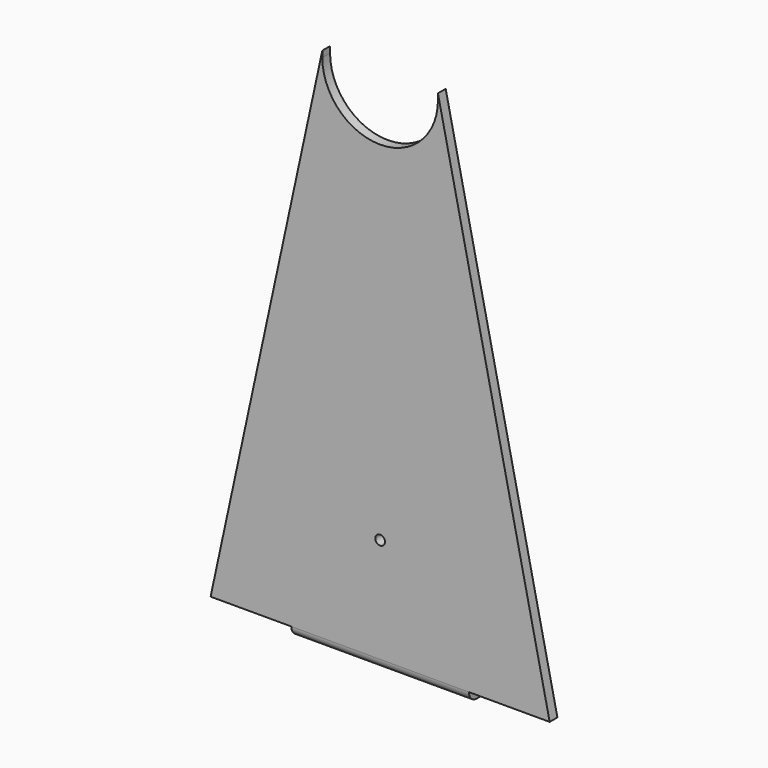
from build123d import *

# Parameters (mm, degrees)
F0_R     = 1.5
F1_DEPTH = 3
F2_W     = 55
F2_H     = 3
F3_DEPTH = 25
F4_R     = 3
F6_DEPTH = 163.1321276775


with BuildPart() as f1:
    # F0 (on Front) → F1 (new body)
    with BuildSketch(Plane.XZ):
        with BuildLine():
            Line((454.8277321524, 574.7700988736), (454.8277321524, 576.6820907487))
            Line((454.8277321524, 576.6820907487), (420.231500864, 416.5509630712))
            Line((420.231500864, 416.5509630712), (495.9500458773, 416.5509630712))
            Line((495.9500458773, 416.5509630712), (525.231500864, 416.5509630712))
            Line((525.231500864, 416.5509630712), (490.6352695757, 576.6820907487))
            Line((490.6352695757, 576.6820907487), (490.6352695757, 574.7700988736))
            ThreePointArc((490.6352695757, 574.7700988736), (472.731500864, 556.866330162), (454.8277321524, 574.7700988736))
        make_face()
        with Locations((472.731500864, 449.0509630712)):
            Circle(F0_R, mode=Mode.SUBTRACT)
    extrude(amount=F1_DEPTH)

    # F2 (on face) → F3 (join)
    with BuildSketch(Plane.XZ.offset(3)):
        with Locations((472.731500864, 415.0509630712)):
            Rectangle(F2_W, F2_H)
    extrude(amount=-F3_DEPTH)

    # F4
    f4_edges = [f1.edges().sort_by_distance(p)[0] for p in [
        (472.731501, -3, 413.550963),
        (472.731501, 0, 416.550963),
    ]]
    fillet(f4_edges, radius=F4_R)

    # F5 (on face) → F6 (cut, through all)
    with BuildSketch(Plane(origin=(0, 0, 413.5509630712), x_dir=(1, 0, 0), z_dir=(0, 0, -1))):
        with BuildLine():
            Line((475.731500864, -15.5), (475.731500864, -7.5))
            ThreePointArc((475.731500864, -7.5), (472.731500864, -4.5), (469.731500864, -7.5))
            Line((469.731500864, -7.5), (469.731500864, -15.5))
            ThreePointArc((469.731500864, -15.5), (472.731500864, -18.5), (475.731500864, -15.5))
        make_face()
    extrude(amount=-F6_DEPTH, mode=Mode.SUBTRACT)


solid = f1.part
